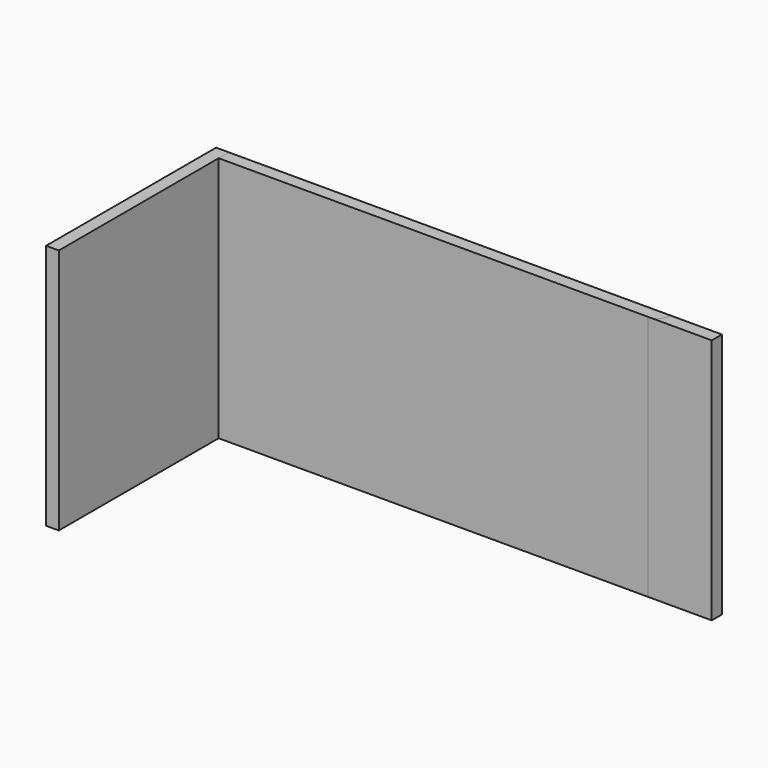
from build123d import *

# Parameters (mm, degrees)
F0_W     = 755.65
F0_H     = 368.3
F1_DEPTH = 19.05
F2_W     = 679.45
F2_H     = 368.3
F3_DEPTH = 19.05
F4_R     = 19.04999
F5_W     = 317.5
F5_H     = 368.3
F6_DEPTH = 19.05


# Not quite as in the source:
# - a fillet or chamfer is up to 0.001 mm smaller than in the source, because OpenCascade refuses the exact size


with BuildPart() as f1:
    # F0 (on Front) → F1 (new body)
    with BuildSketch(Plane.XZ):
        with Locations((377.825, 184.15)):
            Rectangle(F0_W, F0_H)
    extrude(amount=F1_DEPTH)


with BuildPart() as f3:
    # F2 (on Front) → F3 (new body)
    with BuildSketch(Plane.XZ):
        with Locations((339.725, 184.15)):
            Rectangle(F2_W, F2_H)
    extrude(amount=F3_DEPTH)

    # F4 (radius 19.05 in the source; OpenCascade refuses exactly that, so slightly less here)
    f4_edges = [f3.edges().sort_by_distance(p)[0] for p in [
        (679.45, -19.05, 184.15),
    ]]
    fillet(f4_edges, radius=F4_R)


with BuildPart() as f6:
    # F5 (on Right) → F6 (new body)
    with BuildSketch(Plane.YZ):
        with Locations((-158.75, 184.15)):
            Rectangle(F5_W, F5_H)
    extrude(amount=F6_DEPTH)


solid = Compound([f1.part, f3.part, f6.part])
